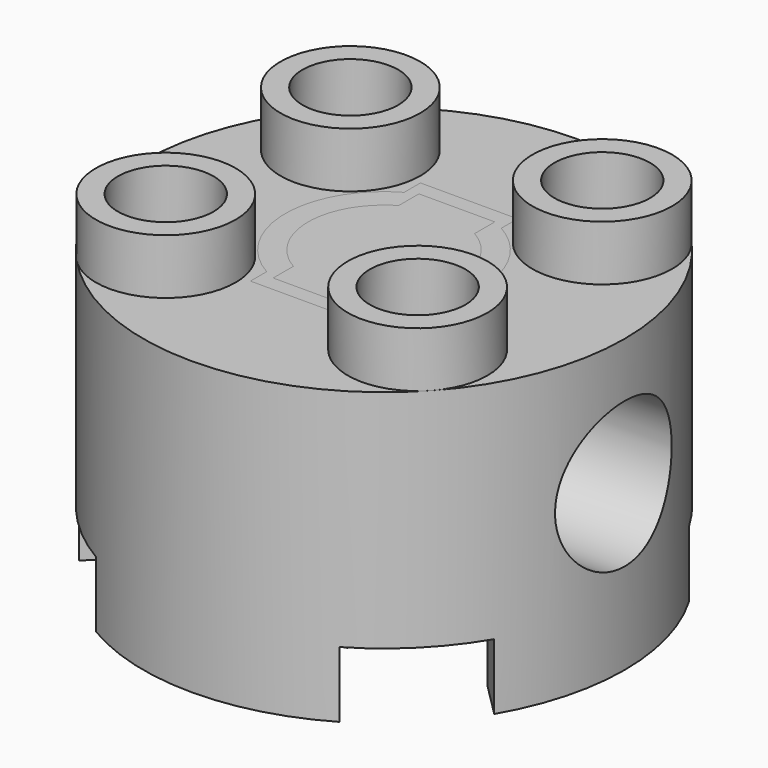
from build123d import *
from build123d import SkipClean  # not in build123d's __all__

# Parameters (mm, degrees)
F0_R      = 7.925
F1_DEPTH  = 9.6
F2_R      = 6.425
F3_DEPTH  = 2.5
F4_R      = 2.3
F4_R_2    = 1.575
F5_DEPTH  = 1.82
F12_W     = 4
F12_H     = 4.34
F13_DEPTH = 22.4162849636
F10_W     = 4
F10_H     = 4.34
F14_DEPTH = 22.4162849636
F17_DEPTH = 9.6
F15_R     = 2.4
F18_DEPTH = 15.851


with BuildPart() as f1:
    # F0 (on Top) → F1 (new body)
    with BuildSketch(Plane.XY):
        Circle(F0_R)
    extrude(amount=F1_DEPTH)

    # F2 (on face) → F3 (cut)
    with BuildSketch(Plane(origin=(0, 0, 0), x_dir=(1, 0, 0), z_dir=(0, 0, -1))):
        Circle(F2_R)
    extrude(amount=-F3_DEPTH, mode=Mode.SUBTRACT)

    # F4 (on face) → F5 (join)
    with BuildSketch(Plane.XY.offset(9.6)):
        with Locations((-4.1473636204, -3.8)):
            Circle(F4_R)
        with Locations((-4.1473636204, -3.8)):
            Circle(F4_R_2, mode=Mode.SUBTRACT)
        with Locations((-4.1473636204, 3.8)):
            Circle(F4_R)
        with Locations((-4.1473636204, 3.8)):
            Circle(F4_R_2, mode=Mode.SUBTRACT)
        with Locations((4.1473636204, 3.8)):
            Circle(F4_R)
        with Locations((4.1473636204, 3.8)):
            Circle(F4_R_2, mode=Mode.SUBTRACT)
        with Locations((4.1473636204, -3.8)):
            Circle(F4_R)
        with Locations((4.1473636204, -3.8)):
            Circle(F4_R_2, mode=Mode.SUBTRACT)
    extrude(amount=F5_DEPTH)

    # F12 (on face) → F13 (cut, through all)
    with BuildSketch(Plane(origin=(7.925, 7.925, 0), x_dir=(-0.7071067812, 0.7071067812, 0), z_dir=(0.7071067812, 0.7071067812, 0))):
        Rectangle(F12_W, F12_H)
    extrude(amount=-F13_DEPTH, mode=Mode.SUBTRACT)

    # F10 (on face) → F14 (cut, through all)
    with BuildSketch(Plane(origin=(7.925, -7.925, 0), x_dir=(0.7071067812, 0.7071067812, 0), z_dir=(0.7071067812, -0.7071067812, 0))):
        Rectangle(F10_W, F10_H)
    extrude(amount=-F14_DEPTH, mode=Mode.SUBTRACT)

    # F16 (on face) → F17 (join)
    with BuildSketch(Plane.XY.offset(9.6)):
        with BuildLine():
            Line((1.6, 2.828869032), (1.6, 3.5))
            Line((1.6, 3.5), (-1.6, 3.5))
            Line((-1.6, 3.5), (-1.6, 2.828869032))
            ThreePointArc((-1.6, 2.828869032), (-1.4275666191, 2.9196838096), (-1.25, 3))
            ThreePointArc((-1.25, 3), (0, 3.25), (1.25, 3))
            ThreePointArc((1.25, 3), (1.4275666191, 2.9196838096), (1.6, 2.828869032))
        make_face()
        with BuildLine():
            ThreePointArc((3.25, 0), (2.8073564077, 1.6374522894), (1.6, 2.828869032))
            Line((1.6, 2.828869032), (1.6, 1.9209372712))
            ThreePointArc((1.6, 1.9209372712), (2.2638462845, 1.0606601718), (2.5, 0))
            ThreePointArc((2.5, 0), (2.2638462845, -1.0606601718), (1.6, -1.9209372712))
            Line((1.6, -1.9209372712), (1.6, -2.828869032))
            ThreePointArc((1.6, -2.828869032), (2.8073564077, -1.6374522894), (3.25, 0))
        make_face()
        with BuildLine():
            Line((1.6, 1.9209372712), (1.6, 2.828869032))
            ThreePointArc((1.6, 2.828869032), (1.4275666191, 2.9196838096), (1.25, 3))
            Line((1.25, 3), (1.25, 2.1650635095))
            ThreePointArc((1.25, 2.1650635095), (1.4302183068, 2.0504817958), (1.6, 1.9209372712))
        make_face()
        with BuildLine():
            ThreePointArc((-1.25, 3), (-1.4275666191, 2.9196838096), (-1.6, 2.828869032))
            Line((-1.6, 2.828869032), (-1.6, 1.9209372712))
            ThreePointArc((-1.6, 1.9209372712), (-1.4302183068, 2.0504817958), (-1.25, 2.1650635095))
            Line((-1.25, 2.1650635095), (-1.25, 3))
        make_face()
        with BuildLine():
            Line((-1.6, 1.9209372712), (-1.6, 2.828869032))
            ThreePointArc((-1.6, 2.828869032), (-3.25, 0), (-1.6, -2.828869032))
            Line((-1.6, -2.828869032), (-1.6, -1.9209372712))
            ThreePointArc((-1.6, -1.9209372712), (-2.5, 0), (-1.6, 1.9209372712))
        make_face()
        with BuildLine():
            ThreePointArc((-1.25, -3), (-1.4275666191, -2.9196838096), (-1.6, -2.828869032))
            Line((-1.6, -2.828869032), (-1.6, -3.5))
            Line((-1.6, -3.5), (1.6, -3.5))
            Line((1.6, -3.5), (1.6, -2.828869032))
            ThreePointArc((1.6, -2.828869032), (1.4275666191, -2.9196838096), (1.25, -3))
            ThreePointArc((1.25, -3), (0, -3.25), (-1.25, -3))
        make_face()
        with BuildLine():
            Line((-1.6, -1.9209372712), (-1.6, -2.828869032))
            ThreePointArc((-1.6, -2.828869032), (-1.4275666191, -2.9196838096), (-1.25, -3))
            Line((-1.25, -3), (-1.25, -2.1650635095))
            ThreePointArc((-1.25, -2.1650635095), (-1.4302183068, -2.0504817958), (-1.6, -1.9209372712))
        make_face()
        with BuildLine():
            Line((1.6, -2.828869032), (1.6, -1.9209372712))
            ThreePointArc((1.6, -1.9209372712), (1.4302183068, -2.0504817958), (1.25, -2.1650635095))
            Line((1.25, -2.1650635095), (1.25, -3))
            ThreePointArc((1.25, -3), (1.4275666191, -2.9196838096), (1.6, -2.828869032))
        make_face()
        with BuildLine():
            Line((-1.25, 3), (1.25, 3))
            ThreePointArc((1.25, 3), (0, 3.25), (-1.25, 3))
        make_face()
        with BuildLine():
            Line((1.25, -3), (-1.25, -3))
            ThreePointArc((-1.25, -3), (0, -3.25), (1.25, -3))
        make_face()
    with SkipClean():  # cleaning this boolean's faces spoils the solid; the shape is the same uncleaned
        extrude(amount=-F17_DEPTH)

    # F15 (on offset) → F18 (cut, through all)
    with BuildSketch(Plane.YZ.offset(7.925)):
        with Locations((0, 5.4)):
            Circle(F15_R)
    with SkipClean():  # cleaning this boolean's faces spoils the solid; the shape is the same uncleaned
        extrude(amount=-F18_DEPTH, mode=Mode.SUBTRACT)


solid = f1.part
